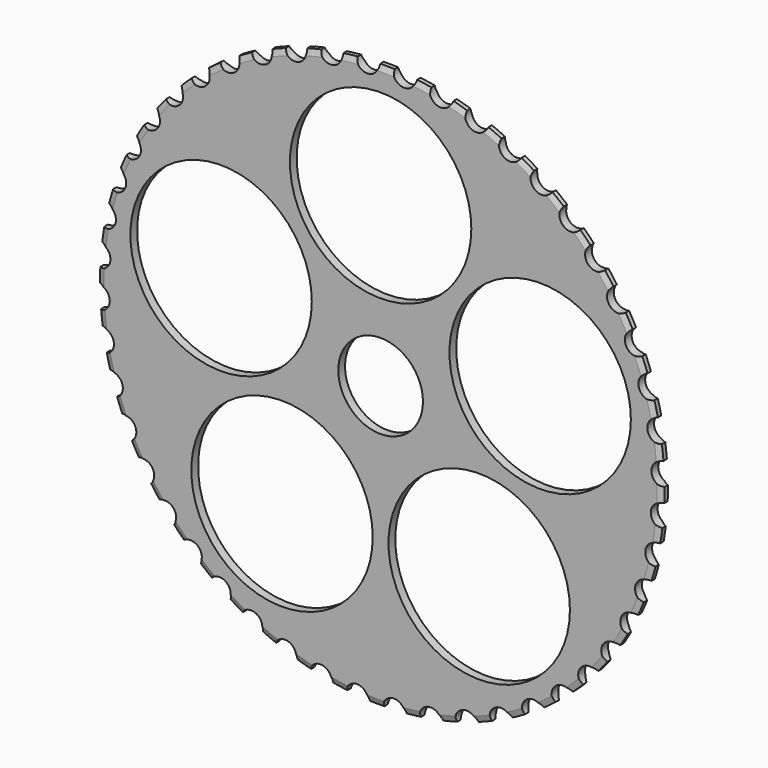
from build123d import *

# Parameters (mm, degrees)
F0_R     = 100
F0_R_2   = 32.1367223505
F1_DEPTH = 3
F2_SIZE2 = 2
F2_SIZE  = 0.75
F4_R     = 4
F4_R_2   = 15
F5_DEPTH = 3.001


# Not quite as in the source:
# - two fillets or chamfers of one size are made in one step


with BuildPart() as f1:
    # F0 (on Front) → F1 (new body)
    with BuildSketch(Plane.XZ):
        Circle(F0_R)
        with Locations((-34.9334680066, -48.0817930464)):
            Circle(F0_R_2, mode=Mode.SUBTRACT)
        with Locations((34.9334673054, -48.0817935558)):
            Circle(F0_R_2, mode=Mode.SUBTRACT)
        with Locations((-56.5235378784, 18.3656112131)):
            Circle(F0_R_2, mode=Mode.SUBTRACT)
        with Locations((56.5235381462, 18.3656103888)):
            Circle(F0_R_2, mode=Mode.SUBTRACT)
        with Locations((4.334e-07, 59.4323650002)):
            Circle(F0_R_2, mode=Mode.SUBTRACT)
    extrude(amount=F1_DEPTH)

    # F2
    f2_edges = [f1.edges().sort_by_distance(p)[0] for p in [
        (-100, 0, 0),
        (-100, -3, 0),
    ]]
    f2_side = f1.faces().sort_by_distance((-100, -1.5, 0))[0]
    chamfer(f2_edges, length=F2_SIZE, length2=F2_SIZE2, reference=f2_side)

    # F4 (on face) → F5 (cut, through all)
    with BuildSketch(Plane.XZ.offset(3)):
        with Locations((-88.9164384293, 45.9052292347)):
            Circle(F4_R)
        with Locations((-94.1475807474, 33.906579501)):
            Circle(F4_R)
        with Locations((-97.7678318562, 21.3277787913)):
            Circle(F4_R)
        with Locations((-99.7152482556, 8.3840538734)):
            Circle(F4_R)
        with Locations((-99.9565091111, -4.7031245308)):
            Circle(F4_R)
        with Locations((-98.4874863826, -17.7098311704)):
            Circle(F4_R)
        with Locations((-95.3333154561, -30.4135176885)):
            Circle(F4_R)
        with Locations((-90.5479650708, -42.5968204868)):
            Circle(F4_R)
        with Locations((-84.2133138984, -54.0512798764)):
            Circle(F4_R)
        with Locations((-76.437749577, -64.5809068816)):
            Circle(F4_R)
        with Locations((-67.3543141677, -74.0055366647)):
            Circle(F4_R)
        with Locations((-57.1184277689, -82.1639111974)):
            Circle(F4_R)
        with Locations((-45.9052292347, -88.9164384293)):
            Circle(F4_R)
        with Locations((-33.906579501, -94.1475807474)):
            Circle(F4_R)
        with Locations((-21.3277787913, -97.7678318562)):
            Circle(F4_R)
        with Locations((-8.3840538734, -99.7152482556)):
            Circle(F4_R)
        with Locations((4.7031245308, -99.9565091111)):
            Circle(F4_R)
        with Locations((17.7098311704, -98.4874863826)):
            Circle(F4_R)
        with Locations((30.4135176885, -95.3333154561)):
            Circle(F4_R)
        with Locations((42.5968204868, -90.5479650708)):
            Circle(F4_R)
        with Locations((54.0512798764, -84.2133138984)):
            Circle(F4_R)
        with Locations((64.5809068816, -76.437749577)):
            Circle(F4_R)
        with Locations((74.0055366647, -67.3543141677)):
            Circle(F4_R)
        with Locations((82.1639111974, -57.1184277689)):
            Circle(F4_R)
        with Locations((88.9164384293, -45.9052292347)):
            Circle(F4_R)
        with Locations((94.1475807474, -33.906579501)):
            Circle(F4_R)
        with Locations((97.7678318562, -21.3277787913)):
            Circle(F4_R)
        with Locations((99.7152482556, -8.3840538734)):
            Circle(F4_R)
        with Locations((99.9565091111, 4.7031245308)):
            Circle(F4_R)
        with Locations((98.4874863826, 17.7098311704)):
            Circle(F4_R)
        with Locations((95.3333154561, 30.4135176885)):
            Circle(F4_R)
        with Locations((90.5479650708, 42.5968204868)):
            Circle(F4_R)
        with Locations((84.2133138984, 54.0512798764)):
            Circle(F4_R)
        with Locations((76.437749577, 64.5809068816)):
            Circle(F4_R)
        with Locations((67.3543141677, 74.0055366647)):
            Circle(F4_R)
        with Locations((57.1184277689, 82.1639111974)):
            Circle(F4_R)
        with Locations((45.9052292347, 88.9164384293)):
            Circle(F4_R)
        with Locations((33.906579501, 94.1475807474)):
            Circle(F4_R)
        with Locations((21.3277787913, 97.7678318562)):
            Circle(F4_R)
        with Locations((8.3840538734, 99.7152482556)):
            Circle(F4_R)
        with Locations((-4.7031245308, 99.9565091111)):
            Circle(F4_R)
        with Locations((-17.7098311704, 98.4874863826)):
            Circle(F4_R)
        with Locations((-30.4135176885, 95.3333154561)):
            Circle(F4_R)
        with Locations((-42.5968204868, 90.5479650708)):
            Circle(F4_R)
        with Locations((-54.0512798764, 84.2133138984)):
            Circle(F4_R)
        with Locations((-64.5809068816, 76.437749577)):
            Circle(F4_R)
        with Locations((-74.0055366647, 67.3543141677)):
            Circle(F4_R)
        with Locations((-82.1639111974, 57.1184277689)):
            Circle(F4_R)
        Circle(F4_R_2)
    extrude(amount=-F5_DEPTH, mode=Mode.SUBTRACT)


solid = f1.part
